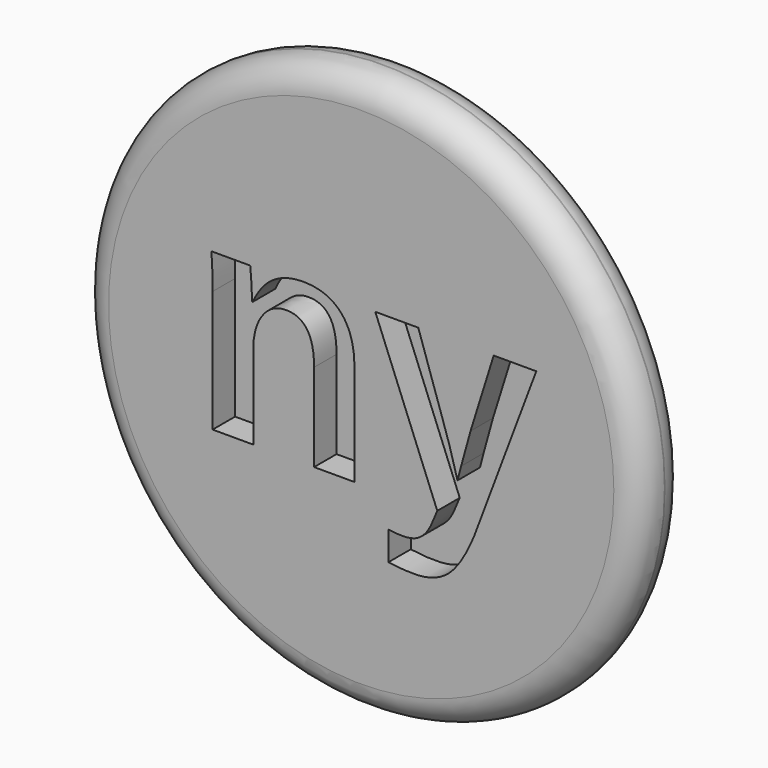
from build123d import *

# Parameters (mm, degrees)
F0_R         = 10
F0_R_2       = 6
F1_DEPTH     = 2.03
F0_R_3       = 4.15
F2_DEPTH     = 2.52
F3_DEPTH     = 6.19
F4_R         = 1
F5_TEXT_SIZE = 10.5610561056
F6_DEPTH     = 1


# Not quite as in the source:
# - a feature names something its author has since deleted; it is built from what else it names
# - Text() gives the source's letters only with a copy of the font that has no kerning and outlines rounded to 1/6400 em; it was checked with that copy


with BuildPart() as f1:
    # F0 (on Front) → F1 (new body)
    with BuildSketch(Plane.XZ):
        Circle(F0_R)
        Circle(F0_R_2, mode=Mode.SUBTRACT)
    extrude(amount=-F1_DEPTH)

    # F0 (on Front) → F2 (join)
    with BuildSketch(Plane.XZ):
        Circle(F0_R_2)
        Circle(F0_R_3, mode=Mode.SUBTRACT)
    extrude(amount=-F2_DEPTH)

    # F0 (on Front) → F3 (join)
    with BuildSketch(Plane.XZ):
        Circle(F0_R_3)
    extrude(amount=-F3_DEPTH)

    # F4
    f4_edges = [f1.edges().sort_by_distance(p)[0] for p in [
        (10, 1.015, 0),
        (-10, 0, 0),
        (-10, 2.03, 0),
    ]]
    fillet(f4_edges, radius=F4_R)

    # F5 (on Front) → F6 (cut)
    with BuildSketch(Plane.XZ):
        with Locations((-6.0312513097, -2.7390196736)):
            Text('ny', F5_TEXT_SIZE, font='Arimo', font_style=FontStyle.BOLD, text_align=(TextAlign.LEFT, TextAlign.BOTTOM))
    extrude(amount=-F6_DEPTH, mode=Mode.SUBTRACT)


solid = f1.part
